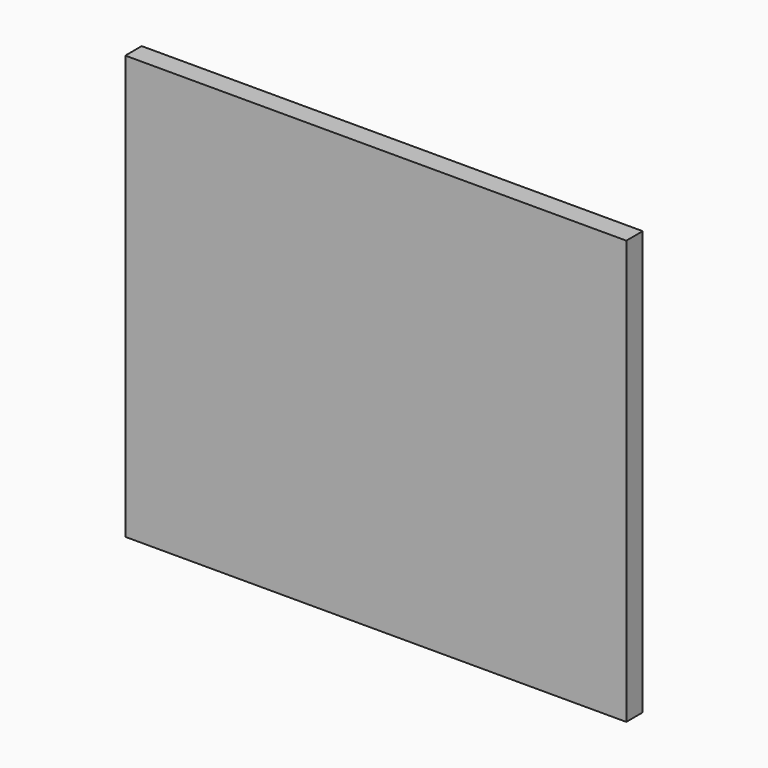
from build123d import *

# Parameters (mm, degrees)
F0_W     = 92.9103940725
F0_H     = 78.5730108619
F1_DEPTH = 3.81


# Not quite as in the source:
# - the program builds the solid bodies; features that only make, move or delete a surface that nothing else refers to are left out


with BuildPart() as f1:
    # F0 (on Front) → F1 (new body)
    with BuildSketch(Plane.XZ):
        with Locations((-9.2773512006, -0.8540265262)):
            Rectangle(F0_W, F0_H)
    extrude(amount=F1_DEPTH)


solid = f1.part
